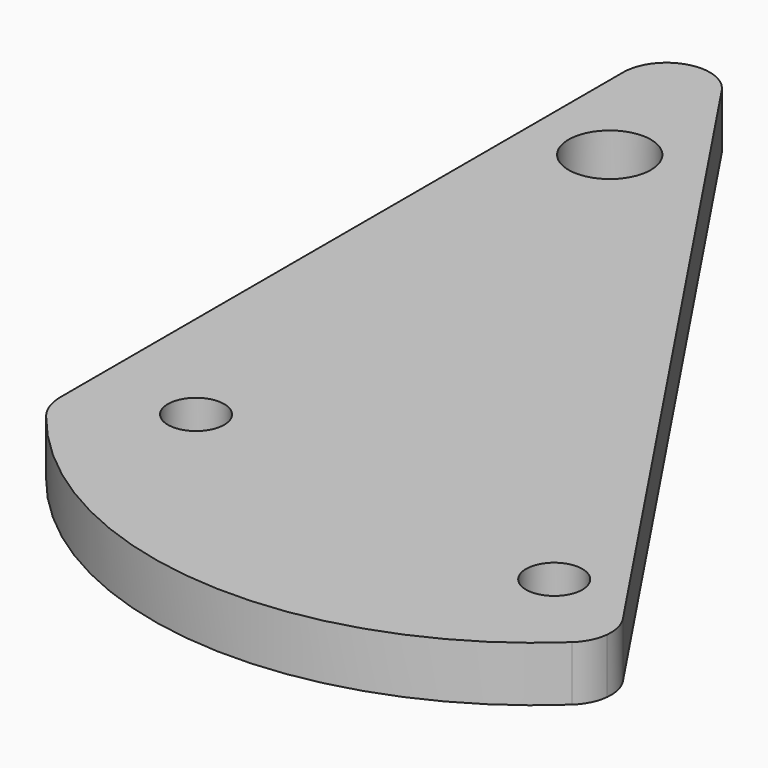
from build123d import *

# Parameters (mm, degrees)
F0_R     = 3.25
F0_R_2   = 4.75
F1_DEPTH = 6.35


# Not quite as in the source:
# - a length typed as a fraction of an inch, garbled in the dataset ("3 / 203.2 mm" for 3/8 in), is restored


with BuildPart() as f1:
    # F0 (on Top) → F1 (new body)
    with BuildSketch(Plane.XY):
        with BuildLine():
            ThreePointArc((-22.8971660057, 33.6711986684), (-28.5061254625, 35.6804376948), (-32.0558722278, 30.8953812108))
            Line((-32.0558722278, 30.8953812108), (-32.0558722278, -50.2885361405))
            ThreePointArc((-32.0558722278, -50.2885361405), (-31.9678509198, -51.3125029104), (-31.7063695792, -52.3064260488))
            Line((-31.7063695792, -52.3064260488), (35.4015681706, -55.732164864))
            ThreePointArc((35.4015681706, -55.732164864), (35.2797878973, -54.0198372397), (34.5860178433, -52.4496208725))
            Line((34.5860178433, -52.4496208725), (-22.8971660057, 33.6711986684))
        make_face()
        with Locations((-20.3956849873, -45.3237444162)):
            Circle(F0_R, mode=Mode.SUBTRACT)
        with Locations((24.9280557036, -50.2885361405)):
            Circle(F0_R, mode=Mode.SUBTRACT)
        with Locations((-22.9451451451, 17.56295003)):
            Circle(F0_R_2, mode=Mode.SUBTRACT)
        with BuildLine():
            Line((35.4015681706, -55.732164864), (-31.7063695792, -52.3064260488))
            ThreePointArc((-31.7063695792, -52.3064260488), (-31.3042287593, -53.1962420607), (-30.763080876, -54.0090450764))
            ThreePointArc((-30.763080876, -54.0090450764), (0.4708891197, -70.6124039736), (33.840882919, -58.8788656243))
            ThreePointArc((33.840882919, -58.8788656243), (34.9066358356, -57.4470716441), (35.4015681706, -55.732164864))
        make_face()
    extrude(amount=F1_DEPTH)


solid = f1.part
